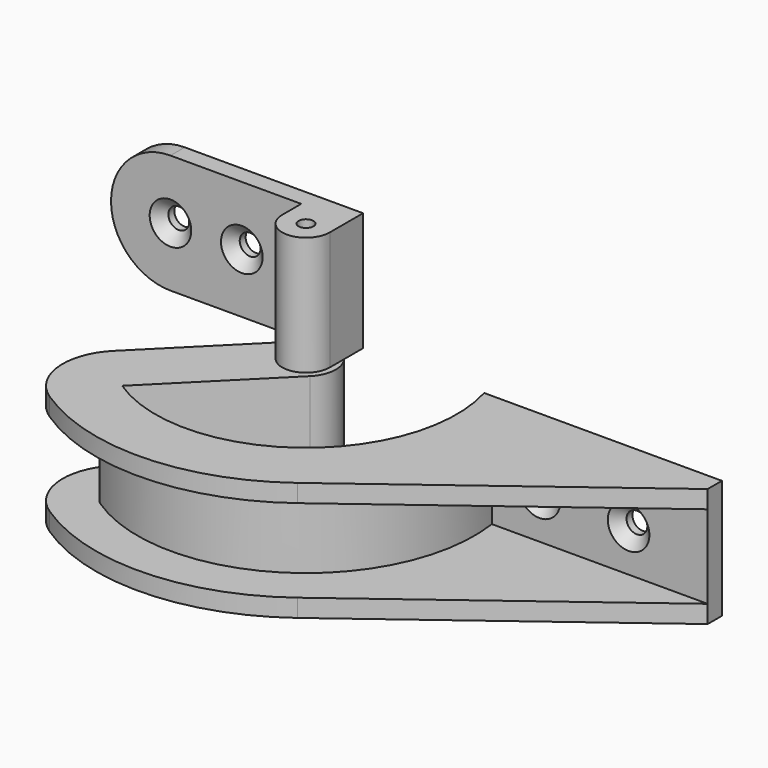
from build123d import *

# Parameters (mm, degrees)
F0_R             = 1.25
F2_DEPTH         = 20
F1_R             = 1.25
F3_DEPTH         = 20
F4_START         = -3
F4_DEPTH         = 14
F5_R             = 9.99999
F5_2_R           = 9.99999
F6_R             = 3
F8_D             = 3.5
F8_DEPTH         = 20
F8_CSINK_D       = 7
F8_CSINK_ANGLE   = 90
F8_TIP           = 1.0515060833
F8_2_D           = 3.5
F8_2_DEPTH       = 20
F8_2_CSINK_D     = 7
F8_2_CSINK_ANGLE = 90
F8_2_TIP         = 1.0515060833


# Not quite as in the source:
# - a fillet or chamfer is up to 0.001 mm smaller than in the source, because OpenCascade refuses the exact size


with BuildPart() as f2:
    # F0 (on Top) → F2 (new body)
    with BuildSketch(Plane.XY):
        with BuildLine():
            Line((4, 7), (-36, 7))
            Line((-36, 7), (-36, 4))
            Line((-36, 4), (-4, 4))
            Line((-4, 4), (-4, 0))
            ThreePointArc((-4, 0), (0, -4), (4, 0))
            Line((4, 0), (4, 7))
        make_face()
        Circle(F0_R, mode=Mode.SUBTRACT)
    extrude(amount=F2_DEPTH)

    # F5 (radius 10 in the source; OpenCascade refuses exactly that, so slightly less here)
    f5_edges = [f2.edges().sort_by_distance(p)[0] for p in [
        (-36, 5.5, 20),
        (-36, 5.5, 0),
    ]]
    fillet(f5_edges, radius=F5_R)

    # F8
    with Locations(Plane.XZ.offset(-4)):
        with Locations((-26, 10), (-14, 10), (36.0717874951, -10), (51.0717874951, -10)):
            CounterSinkHole(F8_D / 2, F8_CSINK_D / 2, depth=F8_DEPTH, counter_sink_angle=F8_CSINK_ANGLE)
            with Locations((0, 0, -(F8_DEPTH + F8_TIP / 2))):  # 118° drill point
                Cone(0, F8_D / 2, F8_TIP, mode=Mode.SUBTRACT)


with BuildPart() as f3:
    # F1 (on Top) → F3 (new body)
    with BuildSketch(Plane.XY):
        with BuildLine():
            Line((-14.0413432173, -21.1124110292), (3.5355339059, -3.5355339059))
            ThreePointArc((3.5355339059, -3.5355339059), (3.5355339059, 3.5355339059), (-3.5355339059, 3.5355339059))
            ThreePointArc((-3.5355339059, 3.5355339059), (-3.9904772202, 3.0126552334), (-4.3687434308, 2.4318883272))
            Line((-4.3687434308, 2.4318883272), (-17.9440420579, -21.9553321039))
            ThreePointArc((-17.9440420579, -21.9553321039), (13.9306361328, -24.6974215274), (28.0717874951, 4))
            Line((28.0717874951, 4), (64.3699244729, 4))
            Line((64.3699244729, 4), (64.3699244729, 7))
            Line((64.3699244729, 7), (24.3699244729, 7))
            ThreePointArc((24.3699244729, 7), (14.9748726591, -20.4608506093), (-14.0413432173, -21.1124110292))
        make_face()
        Circle(F1_R, mode=Mode.SUBTRACT)
        with BuildLine():
            ThreePointArc((-4.3687434308, 2.4318883272), (-3.9904772202, 3.0126552334), (-3.5355339059, 3.5355339059))
            Line((-3.5355339059, 3.5355339059), (-28.2842712475, -21.2132034356))
            ThreePointArc((-28.2842712475, -21.2132034356), (-5.0216203507, -34.9969045639), (21.1782419461, -28.3104586341))
            Line((21.1782419461, -28.3104586341), (64.3699244729, 4))
            Line((64.3699244729, 4), (28.0717874951, 4))
            ThreePointArc((28.0717874951, 4), (13.9306361328, -24.6974215274), (-17.9440420579, -21.9553321039))
            Line((-17.9440420579, -21.9553321039), (-4.3687434308, 2.4318883272))
        make_face()
    extrude(amount=-F3_DEPTH)

    # F1 (on Top) → F4 (cut)
    with BuildSketch(Plane.XY.offset(F4_START)):
        with BuildLine():
            ThreePointArc((-4.3687434308, 2.4318883272), (-3.9904772202, 3.0126552334), (-3.5355339059, 3.5355339059))
            Line((-3.5355339059, 3.5355339059), (-28.2842712475, -21.2132034356))
            ThreePointArc((-28.2842712475, -21.2132034356), (-5.0216203507, -34.9969045639), (21.1782419461, -28.3104586341))
            Line((21.1782419461, -28.3104586341), (64.3699244729, 4))
            Line((64.3699244729, 4), (28.0717874951, 4))
            ThreePointArc((28.0717874951, 4), (13.9306361328, -24.6974215274), (-17.9440420579, -21.9553321039))
            Line((-17.9440420579, -21.9553321039), (-4.3687434308, 2.4318883272))
        make_face()
    extrude(amount=-F4_DEPTH, mode=Mode.SUBTRACT)

    # F5#2 (radius 10 in the source; OpenCascade refuses exactly that, so slightly less here)
    f5_2_edges = [f3.edges().sort_by_distance(p)[0] for p in [
        (-28.284271, -21.213203, -1.5),
        (-28.284271, -21.213203, -18.5),
    ]]
    fillet(f5_2_edges, radius=F5_2_R)

    # F6
    f6_edges = [f3.edges().sort_by_distance(p)[0] for p in [
        (-17.944042, -21.955332, -10),
    ]]
    fillet(f6_edges, radius=F6_R)

    # F8#2
    with Locations(Plane.XZ.offset(-4)):
        with Locations((-26, 10), (-14, 10), (36.0717874951, -10), (51.0717874951, -10)):
            CounterSinkHole(F8_2_D / 2, F8_2_CSINK_D / 2, depth=F8_2_DEPTH, counter_sink_angle=F8_2_CSINK_ANGLE)
            with Locations((0, 0, -(F8_2_DEPTH + F8_2_TIP / 2))):  # 118° drill point
                Cone(0, F8_2_D / 2, F8_2_TIP, mode=Mode.SUBTRACT)


solid = Compound([f2.part, f3.part])
